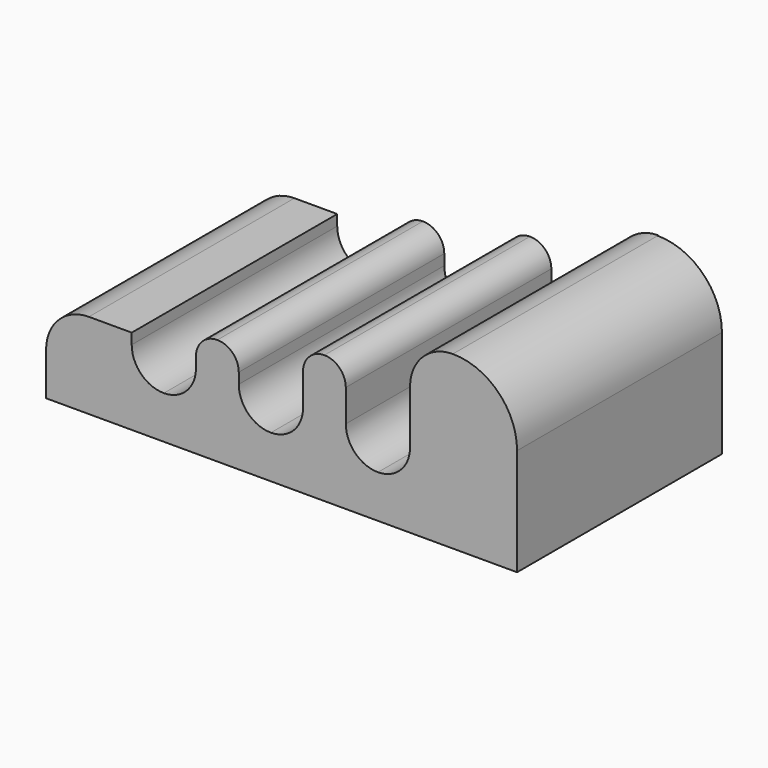
from build123d import *

# Parameters (mm, degrees)
F0_W      = 12.7
F0_H      = 25.4
F0_W_2    = 25.4
F1_DEPTH  = 152.4
F2_W      = 152.4
F2_H      = 25.4
F3_DEPTH  = 38.1
F4_R      = 25.4
F6_DEPTH  = 151.892
F7_R      = 19.05
F8_R      = 19.04999
F9_R      = 19.04999
F10_R     = 12.69999
F11_R     = 25.39999
F12_ANGLE = 90


# Not quite as in the source:
# - a fillet or chamfer is up to 0.001 mm smaller than in the source, because OpenCascade refuses the exact size


with BuildPart() as f1:
    # F0 (on Front) → F1 (new body)
    with BuildSketch(Plane.XZ):
        Polygon((-147.5200289965, 215.9), (-172.9200289965, 215.9), (-249.1200289965, 215.9), (-249.1200289965, 190.5), (-172.9200289965, 190.5), (-172.9200289965, 152.4), (-223.7200289965, 152.4), (-223.7200289965, 127), (-172.9200289965, 127), (-172.9200289965, 88.9), (-211.0200289965, 88.9), (-211.0200289965, 63.5), (-172.9200289965, 63.5), (-172.9200289965, 25.4), (-172.9200289965, 0), (-160.2200289965, 0), (-147.5200289965, 0), (-147.5200289965, 63.5), (-147.5200289965, 88.9), (-147.5200289965, 127), (-147.5200289965, 152.4), (-147.5200289965, 190.5), align=None)
        with Locations((-153.8700289965, -12.7)):
            Rectangle(F0_W, F0_H)
        with Locations((-185.6200289965, 12.7)):
            Rectangle(F0_W_2, F0_H)
    extrude(amount=F1_DEPTH)

    # F2 (on face) → F3 (join)
    with BuildSketch(Plane(origin=(-160.2200289965, 0, 0), x_dir=(0, -1, 0), z_dir=(-1, 0, 0))):
        with Locations((76.2, -12.7)):
            Rectangle(F2_W, F2_H)
    extrude(amount=F3_DEPTH)

    # F4
    f4_edges = [f1.edges().sort_by_distance(p)[0] for p in [
        (-198.320029, -76.2, -25.4),
    ]]
    fillet(f4_edges, radius=F4_R)

    # F5 (on face) → F6 (join)
    with BuildSketch(Plane.XZ.offset(152.4)):
        with BuildLine():
            ThreePointArc((-211.0200289965, 254), (-237.9607973597, 242.8407683632), (-249.1200289965, 215.9))
            Line((-249.1200289965, 215.9), (-147.5200289965, 215.9))
            Line((-147.5200289965, 215.9), (-147.5200289965, 254))
            Line((-147.5200289965, 254), (-211.0200289965, 254))
        make_face()
    extrude(amount=-F6_DEPTH)

    # F7
    f7_edges = [f1.edges().sort_by_distance(p)[0] for p in [
        (-172.920029, -76.2, 88.9),
    ]]
    fillet(f7_edges, radius=F7_R)

    # F8 (radius 19.05 in the source; OpenCascade refuses exactly that, so slightly less here)
    f8_edges = [f1.edges().sort_by_distance(p)[0] for p in [
        (-172.920029, -76.2, 190.5),
        (-172.920029, -76.2, 127),
    ]]
    fillet(f8_edges, radius=F8_R)

    # F9 (radius 19.05 in the source; OpenCascade refuses exactly that, so slightly less here)
    f9_edges = [f1.edges().sort_by_distance(p)[0] for p in [
        (-172.920029, -76.2, 152.4),
        (-172.920029, -76.2, 25.4),
        (-172.920029, -76.2, 63.5),
    ]]
    fillet(f9_edges, radius=F9_R)

    # F10 (radius 12.7 in the source; OpenCascade refuses exactly that, so slightly less here)
    f10_edges = [f1.edges().sort_by_distance(p)[0] for p in [
        (-223.720029, -76.2, 152.4),
        (-223.720029, -76.2, 127),
        (-211.020029, -76.2, 88.9),
        (-211.020029, -76.2, 63.5),
    ]]
    fillet(f10_edges, radius=F10_R)

    # F11 (radius 25.4 in the source; OpenCascade refuses exactly that, so slightly less here)
    f11_edges = [f1.edges().sort_by_distance(p)[0] for p in [
        (-249.120029, -76.2, 190.5),
    ]]
    fillet(f11_edges, radius=F11_R)


with BuildPart() as f1_1:
    # F12: moved
    add(f1.part.rotate(Axis((-147.5200289965, -76.2, -25.4), (0, 1, 0)), F12_ANGLE))


solid = f1_1.part
